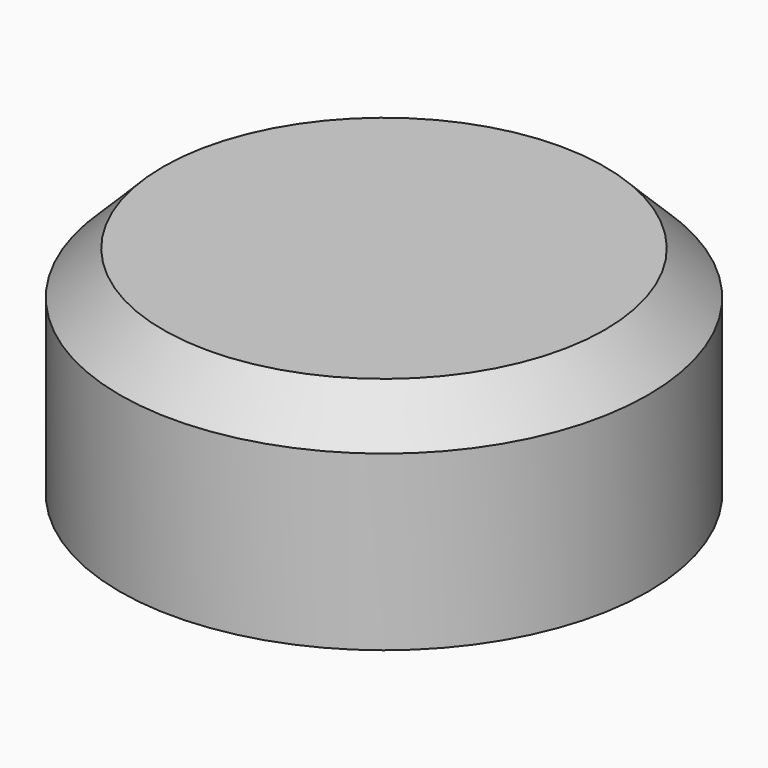
from build123d import *

# Parameters (mm, degrees)
F0_R     = 30.5145931063
F1_DEPTH = 25
F4_SIZE  = 5


# Not quite as in the source:
# - the program builds the solid bodies; features that only make, move or delete a surface that nothing else refers to are left out


with BuildPart() as f1:
    # F0 (on Top) → F1 (new body)
    with BuildSketch(Plane.XY):
        with Locations((-38.9882139862, 42.7013747394)):
            Circle(F0_R)
    extrude(amount=F1_DEPTH)

    # F4
    f4_edges = [f1.edges().sort_by_distance(p)[0] for p in [
        (-69.502807, 42.701375, 25),
    ]]
    chamfer(f4_edges, length=F4_SIZE)


solid = f1.part
